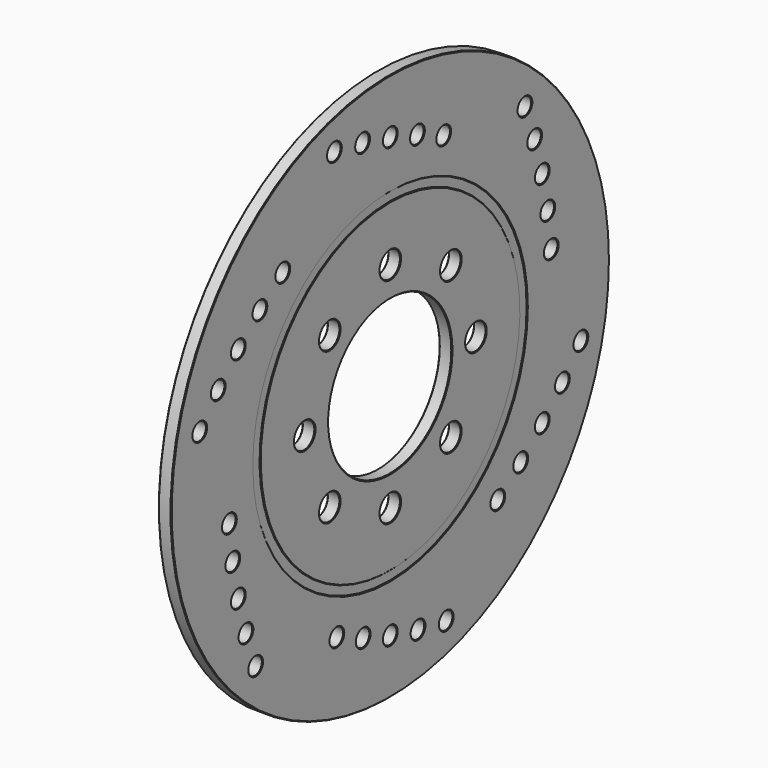
from build123d import *

# Parameters (mm, degrees)
F0_R     = 101.6
F0_R_2   = 3.175
F0_R_3   = 4.7625
F0_R_4   = 28.575
F1_DEPTH = 2.38125
F2_W     = 23.27275
F2_H     = 3.175
F4_SIZE  = 0.25399


# Not quite as in the source:
# - a fillet or chamfer is up to 0.001 mm smaller than in the source, because OpenCascade refuses the exact size


with BuildPart() as f1:
    # F0 (on Right) → F1 (new body, symmetric)
    with BuildSketch(Plane.YZ):
        Circle(F0_R)
        with Locations((-62.4282468049, -65.9764627324)):
            Circle(F0_R_2, mode=Mode.SUBTRACT)
        with Locations((-66.9177945797, -53.478147823)):
            Circle(F0_R_2, mode=Mode.SUBTRACT)
        with Locations((-12.5679149295, -77.0653458753)):
            Circle(F0_R_2, mode=Mode.SUBTRACT)
        with Locations((0, -81.3562)):
            Circle(F0_R_2, mode=Mode.SUBTRACT)
        with Locations((-24.7782971774, -71.843231346)):
            Circle(F0_R_2, mode=Mode.SUBTRACT)
        with Locations((-70.4565359554, -40.6781)):
            Circle(F0_R_2, mode=Mode.SUBTRACT)
        with Locations((-73.0245047442, -27.6485393361)):
            Circle(F0_R_2, mode=Mode.SUBTRACT)
        with Locations((-74.6072120243, -14.4629808549)):
            Circle(F0_R_2, mode=Mode.SUBTRACT)
        with Locations((-28.0633003783, -28.0633003783)):
            Circle(F0_R_3, mode=Mode.SUBTRACT)
        with Locations((0, -39.6875)):
            Circle(F0_R_3, mode=Mode.SUBTRACT)
        with Locations((-39.6875, 0)):
            Circle(F0_R_3, mode=Mode.SUBTRACT)
        Circle(F0_R_4, mode=Mode.SUBTRACT)
        with Locations((12.8545372722, -84.6915839827)):
            Circle(F0_R_2, mode=Mode.SUBTRACT)
        with Locations((25.9231693756, -87.052679013)):
            Circle(F0_R_2, mode=Mode.SUBTRACT)
        with Locations((49.8289148469, -57.3802504911)):
            Circle(F0_R_2, mode=Mode.SUBTRACT)
        with Locations((28.0633003783, -28.0633003783)):
            Circle(F0_R_3, mode=Mode.SUBTRACT)
        with Locations((39.6875, 0)):
            Circle(F0_R_3, mode=Mode.SUBTRACT)
        with Locations((60.4565898147, -49.4168065392)):
            Circle(F0_R_2, mode=Mode.SUBTRACT)
        with Locations((70.4565359554, -40.6781)):
            Circle(F0_R_2, mode=Mode.SUBTRACT)
        with Locations((79.7723318519, -31.2134361597)):
            Circle(F0_R_2, mode=Mode.SUBTRACT)
        with Locations((88.3514161805, -21.0762162806)):
            Circle(F0_R_2, mode=Mode.SUBTRACT)
        with Locations((-88.3514161805, 21.0762162806)):
            Circle(F0_R_2, mode=Mode.SUBTRACT)
        with Locations((-79.7723318519, 31.2134361597)):
            Circle(F0_R_2, mode=Mode.SUBTRACT)
        with Locations((-70.4565359554, 40.6781)):
            Circle(F0_R_2, mode=Mode.SUBTRACT)
        with Locations((-60.4565898147, 49.4168065392)):
            Circle(F0_R_2, mode=Mode.SUBTRACT)
        with Locations((-28.0633003783, 28.0633003783)):
            Circle(F0_R_3, mode=Mode.SUBTRACT)
        with Locations((0, 39.6875)):
            Circle(F0_R_3, mode=Mode.SUBTRACT)
        with Locations((-49.8289148469, 57.3802504911)):
            Circle(F0_R_2, mode=Mode.SUBTRACT)
        with Locations((-25.9231693756, 87.052679013)):
            Circle(F0_R_2, mode=Mode.SUBTRACT)
        with Locations((-12.8545372722, 84.6915839827)):
            Circle(F0_R_2, mode=Mode.SUBTRACT)
        with Locations((0, 81.3562)):
            Circle(F0_R_2, mode=Mode.SUBTRACT)
        with Locations((28.0633003783, 28.0633003783)):
            Circle(F0_R_3, mode=Mode.SUBTRACT)
        with Locations((74.6072120243, 14.4629808549)):
            Circle(F0_R_2, mode=Mode.SUBTRACT)
        with Locations((73.0245047442, 27.6485393361)):
            Circle(F0_R_2, mode=Mode.SUBTRACT)
        with Locations((70.4565359554, 40.6781)):
            Circle(F0_R_2, mode=Mode.SUBTRACT)
        with Locations((24.7782971774, 71.843231346)):
            Circle(F0_R_2, mode=Mode.SUBTRACT)
        with Locations((12.5679149295, 77.0653458753)):
            Circle(F0_R_2, mode=Mode.SUBTRACT)
        with Locations((66.9177945797, 53.478147823)):
            Circle(F0_R_2, mode=Mode.SUBTRACT)
        with Locations((62.4282468049, 65.9764627324)):
            Circle(F0_R_2, mode=Mode.SUBTRACT)
    extrude(amount=F1_DEPTH, both=True)

    # F2 (on Front) → F3 (revolve, cut)
    with BuildSketch(Plane.XZ):
        with Locations((-13.763625, 61.9125)):
            Rectangle(F2_W, F2_H)
        with Locations((13.763625, 61.9125)):
            Rectangle(F2_W, F2_H)
    revolve(axis=Axis((-12.7, 0, 0), (-1, 0, 0)), mode=Mode.SUBTRACT)

    # F4 (size 0.254 in the source; OpenCascade refuses exactly that, so slightly less here)
    f4_edges = [f1.edges().sort_by_distance(p)[0] for p in [
        (-2.38125, -101.6, 0),
        (-2.38125, -65.603247, -65.976463),
        (-2.38125, -70.092795, -53.478148),
        (-2.38125, -27.953297, -71.843231),
        (-2.38125, -3.175, -81.3562),
        (-2.38125, -15.742915, -77.065346),
        (-2.38125, -73.631536, -40.6781),
        (-2.38125, -76.199505, -27.648539),
        (-2.38125, -77.782212, -14.462981),
        (-2.38125, 9.679537, -84.691584),
        (-2.38125, 22.748169, -87.052679),
        (-2.38125, 46.653915, -57.38025),
        (-2.38125, 57.28159, -49.416807),
        (-2.38125, 67.281536, -40.6781),
        (-2.38125, 76.597332, -31.213436),
        (-2.38125, 85.176416, -21.076216),
        (-2.38125, -91.526416, 21.076216),
        (-2.38125, -82.947332, 31.213436),
        (-2.38125, -73.631536, 40.6781),
        (-2.38125, 0, -63.5),
        (-2.38125, -63.63159, 49.416807),
        (-2.38125, -53.003915, 57.38025),
        (-2.38125, -29.098169, 87.052679),
        (-2.38125, -16.029537, 84.691584),
        (-2.38125, -3.175, 81.3562),
        (-2.38125, 71.432212, 14.462981),
        (-2.38125, 69.849505, 27.648539),
        (-2.38125, 67.281536, 40.6781),
        (-2.38125, 9.392915, 77.065346),
        (-2.38125, 21.603297, 71.843231),
        (-2.38125, 63.742795, 53.478148),
        (-2.38125, 59.253247, 65.976463),
        (-2.38125, 0, -60.325),
        (-2.38125, -32.8258, -28.0633),
        (-2.38125, -4.7625, -39.6875),
        (-2.38125, 23.3008, -28.0633),
        (-2.38125, -44.45, 0),
        (-2.38125, -28.575, 0),
        (-2.38125, -32.8258, 28.0633),
        (-2.38125, -4.7625, 39.6875),
        (-2.38125, 34.925, 0),
        (-2.38125, 23.3008, 28.0633),
        (2.38125, 0, -60.325),
        (2.38125, -32.8258, -28.0633),
        (2.38125, -4.7625, -39.6875),
        (2.38125, 23.3008, -28.0633),
        (2.38125, -44.45, 0),
        (2.38125, -28.575, 0),
        (2.38125, -32.8258, 28.0633),
        (2.38125, -4.7625, 39.6875),
        (2.38125, 34.925, 0),
        (2.38125, 23.3008, 28.0633),
        (2.38125, -101.6, 0),
        (2.38125, -65.603247, -65.976463),
        (2.38125, -70.092795, -53.478148),
        (2.38125, -27.953297, -71.843231),
        (2.38125, -3.175, -81.3562),
        (2.38125, -15.742915, -77.065346),
        (2.38125, -73.631536, -40.6781),
        (2.38125, -76.199505, -27.648539),
        (2.38125, -77.782212, -14.462981),
        (2.38125, 9.679537, -84.691584),
        (2.38125, 22.748169, -87.052679),
        (2.38125, 46.653915, -57.38025),
        (2.38125, 57.28159, -49.416807),
        (2.38125, 67.281536, -40.6781),
        (2.38125, 76.597332, -31.213436),
        (2.38125, 85.176416, -21.076216),
        (2.38125, -91.526416, 21.076216),
        (2.38125, -82.947332, 31.213436),
        (2.38125, -73.631536, 40.6781),
        (2.38125, 0, -63.5),
        (2.38125, -63.63159, 49.416807),
        (2.38125, -53.003915, 57.38025),
        (2.38125, -29.098169, 87.052679),
        (2.38125, -16.029537, 84.691584),
        (2.38125, -3.175, 81.3562),
        (2.38125, 71.432212, 14.462981),
        (2.38125, 69.849505, 27.648539),
        (2.38125, 67.281536, 40.6781),
        (2.38125, 9.392915, 77.065346),
        (2.38125, 21.603297, 71.843231),
        (2.38125, 63.742795, 53.478148),
        (2.38125, 59.253247, 65.976463),
    ]]
    chamfer(f4_edges, length=F4_SIZE)


solid = f1.part
